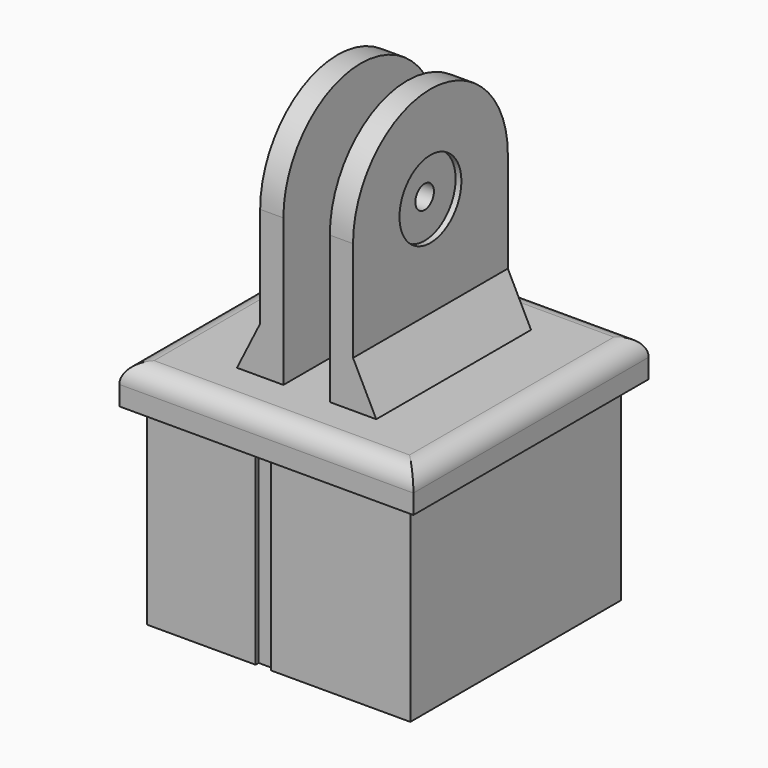
from build123d import *

# Parameters (mm, degrees)
F0_W      = 38
F0_H      = 38
F0_W_2    = 34
F0_H_2    = 34
F0_W_3    = 30
F0_H_3    = 30
F1_DEPTH  = 5
F2_DEPTH  = 25
F4_DEPTH  = 25
F5_DEPTH  = 25
F6_R      = 2.5
F7_W      = 3
F7_H      = 25
F8_DEPTH  = 19
F9_DEPTH  = 19
F10_DEPTH = 6
F11_SIZE2 = 5.99999
F11_SIZE  = 2.99999
F12_SIZE2 = 2.99999
F12_SIZE  = 5.99999
F14_DEPTH = 3
F16_DEPTH = 3
F17_D     = 3
F18_DEPTH = 0.75
F19_DEPTH = 3
F20_DEPTH = 1.5
F21_W     = 2
F21_H     = 25
F22_DEPTH = 0.5


# Not quite as in the source:
# - a fillet or chamfer is up to 0.001 mm smaller than in the source, because OpenCascade refuses the exact size
# - a feature names something its author has since deleted; it is built from what else it names


with BuildPart() as f1:
    # F0 (on Top) → F1 (new body)
    with BuildSketch(Plane.XY):
        Rectangle(F0_W, F0_H)
        Rectangle(F0_W_2, F0_H_2, mode=Mode.SUBTRACT)
        Rectangle(F0_W_2, F0_H_2)
        Rectangle(F0_W_3, F0_H_3, mode=Mode.SUBTRACT)
        Rectangle(F0_W_3, F0_H_3)
    extrude(amount=F1_DEPTH)

    # F0 (on Top) → F2 (join)
    with BuildSketch(Plane.XY):
        Rectangle(F0_W_2, F0_H_2)
        Rectangle(F0_W_3, F0_H_3, mode=Mode.SUBTRACT)
    extrude(amount=-F2_DEPTH)

    # F3 (on face) → F4 (join)
    with BuildSketch(Plane.XY):
        Polygon((1.4142135624, 0), (0.7071067812, 0.7071067812), (0, 1.4142135624), (-13.5857864376, 15), (-15, 15), (-15, 13.5857864376), (-1.4142135624, 0), (-0.7071067812, -0.7071067812), (0, -1.4142135624), (13.5857864376, -15), (15, -15), (15, -13.5857864376), align=None)
        Polygon((0, 1.4142135624), (0.7071067812, 0.7071067812), (1.4142135624, 0), (15, 13.5857864376), (15, 15), (13.5857864376, 15), align=None)
    extrude(amount=-F4_DEPTH)

    # F3 (on face) → F5 (join)
    with BuildSketch(Plane.XY):
        Polygon((-0.7071067812, -0.7071067812), (-1.4142135624, 0), (-15, -13.5857864376), (-15, -15), (-13.5857864376, -15), (0, -1.4142135624), align=None)
    extrude(amount=-F5_DEPTH)

    # F6
    f6_edges = [f1.edges().sort_by_distance(p)[0] for p in [
        (0, 19, 5),
        (19, 0, 5),
        (-19, 0, 5),
        (0, -19, 5),
    ]]
    fillet(f6_edges, radius=F6_R)

    # F7 (on face) → F8 (join)
    with BuildSketch(Plane.XY.offset(5)):
        with Locations((-4.5, 0)):
            Rectangle(F7_W, F7_H)
    extrude(amount=F8_DEPTH)

    # F7 (on face) → F9 (join)
    with BuildSketch(Plane.XY.offset(5)):
        with Locations((4.5, 0)):
            Rectangle(F7_W, F7_H)
    extrude(amount=F9_DEPTH)

    # F7 (on face) → F10 (join)
    with BuildSketch(Plane.XY.offset(5)):
        with Locations((-7.5, 0)):
            Rectangle(F7_W, F7_H)
        with Locations((7.5, 0)):
            Rectangle(F7_W, F7_H)
    extrude(amount=F10_DEPTH)

    # F11 (size 3 and 6 in the source; OpenCascade refuses exactly that, so slightly less here)
    f11_edges = [f1.edges().sort_by_distance(p)[0] for p in [
        (-9, 0, 11),
    ]]
    f11_side = f1.faces().sort_by_distance((-7.5, 0, 11))[0]
    chamfer(f11_edges, length=F11_SIZE, length2=F11_SIZE2, reference=f11_side)

    # F12 (size 6 and 3 in the source; OpenCascade refuses exactly that, so slightly less here)
    f12_edges = [f1.edges().sort_by_distance(p)[0] for p in [
        (9, 0, 11),
    ]]
    f12_side = f1.faces().sort_by_distance((9, 0, 8))[0]
    chamfer(f12_edges, length=F12_SIZE, length2=F12_SIZE2, reference=f12_side)

    # F13 (on face) → F14 (join)
    with BuildSketch(Plane.YZ.offset(6)):
        with BuildLine():
            ThreePointArc((-12.5, 24), (0, 11.5), (12.5, 24))
            Line((12.5, 24), (5, 24))
            ThreePointArc((5, 24), (0, 19), (-5, 24))
            Line((-5, 24), (-12.5, 24))
        make_face()
        with BuildLine():
            Line((5, 24), (12.5, 24))
            ThreePointArc((12.5, 24), (0, 36.5), (-12.5, 24))
            Line((-12.5, 24), (-5, 24))
            ThreePointArc((-5, 24), (0, 29), (5, 24))
        make_face()
        with BuildLine():
            Line((1.5, 24), (5, 24))
            ThreePointArc((5, 24), (0, 29), (-5, 24))
            Line((-5, 24), (-1.5, 24))
            ThreePointArc((-1.5, 24), (0, 25.5), (1.5, 24))
        make_face()
        with BuildLine():
            Line((-1.5, 24), (1.5, 24))
            ThreePointArc((1.5, 24), (0, 25.5), (-1.5, 24))
        make_face()
    extrude(amount=-F14_DEPTH)

    # F15 (on face) → F16 (join)
    with BuildSketch(Plane(origin=(-6, 0, 0), x_dir=(0, -1, 0), z_dir=(-1, 0, 0))):
        with BuildLine():
            Line((-1.5, 24), (1.5, 24))
            ThreePointArc((1.5, 24), (0, 25.5), (-1.5, 24))
        make_face()
    extrude(amount=-F16_DEPTH)

    # F17 (through all)
    with Locations(Plane.YZ.offset(6)):
        with Locations((0, 24)):
            Hole(F17_D / 2)

    # F13 (on face) → F18 (cut, symmetric)
    with BuildSketch(Plane.YZ.offset(6)):
        with BuildLine():
            ThreePointArc((-5, 24), (0, 19), (5, 24))
            Line((5, 24), (1.5, 24))
            ThreePointArc((1.5, 24), (0, 22.5), (-1.5, 24))
            Line((-1.5, 24), (-5, 24))
        make_face()
        with BuildLine():
            Line((1.5, 24), (5, 24))
            ThreePointArc((5, 24), (0, 29), (-5, 24))
            Line((-5, 24), (-1.5, 24))
            ThreePointArc((-1.5, 24), (0, 25.5), (1.5, 24))
        make_face()
    extrude(amount=F18_DEPTH, both=True, mode=Mode.SUBTRACT)

    # F15 (on face) → F19 (join)
    with BuildSketch(Plane(origin=(-6, 0, 0), x_dir=(0, -1, 0), z_dir=(-1, 0, 0))):
        with BuildLine():
            Line((3.5, 24), (12.5, 24))
            ThreePointArc((12.5, 24), (0, 36.5), (-12.5, 24))
            Line((-12.5, 24), (-3.5, 24))
            Line((-3.5, 24), (-3.5, 26.0207259422))
            Line((-3.5, 26.0207259422), (0, 28.0414518843))
            Line((0, 28.0414518843), (3.5, 26.0207259422))
            Line((3.5, 26.0207259422), (3.5, 24))
        make_face()
        with BuildLine():
            Line((1.5, 24), (3.5, 24))
            Line((3.5, 24), (3.5, 26.0207259422))
            Line((3.5, 26.0207259422), (0, 28.0414518843))
            Line((0, 28.0414518843), (-3.5, 26.0207259422))
            Line((-3.5, 26.0207259422), (-3.5, 24))
            Line((-3.5, 24), (-1.5, 24))
            ThreePointArc((-1.5, 24), (0, 25.5), (1.5, 24))
        make_face()
    extrude(amount=-F19_DEPTH)

    # F15 (on face) → F20 (cut)
    with BuildSketch(Plane(origin=(-6, 0, 0), x_dir=(0, -1, 0), z_dir=(-1, 0, 0))):
        with BuildLine():
            Line((1.5, 24), (3.5, 24))
            Line((3.5, 24), (3.5, 26.0207259422))
            Line((3.5, 26.0207259422), (0, 28.0414518843))
            Line((0, 28.0414518843), (-3.5, 26.0207259422))
            Line((-3.5, 26.0207259422), (-3.5, 24))
            Line((-3.5, 24), (-1.5, 24))
            ThreePointArc((-1.5, 24), (0, 25.5), (1.5, 24))
        make_face()
        with BuildLine():
            Line((3.5, 21.9792740578), (3.5, 24))
            Line((3.5, 24), (1.5, 24))
            ThreePointArc((1.5, 24), (0, 22.5), (-1.5, 24))
            Line((-1.5, 24), (-3.5, 24))
            Line((-3.5, 24), (-3.5, 21.9792740578))
            Line((-3.5, 21.9792740578), (0, 19.9585481157))
            Line((0, 19.9585481157), (3.5, 21.9792740578))
        make_face()
    extrude(amount=-F20_DEPTH, mode=Mode.SUBTRACT)

    # F21 (on face) → F22 (cut, symmetric)
    with BuildSketch(Plane.XZ.offset(17)):
        with Locations((-2, -12.5)):
            Rectangle(F21_W, F21_H)
    extrude(amount=F22_DEPTH, both=True, mode=Mode.SUBTRACT)


solid = f1.part
